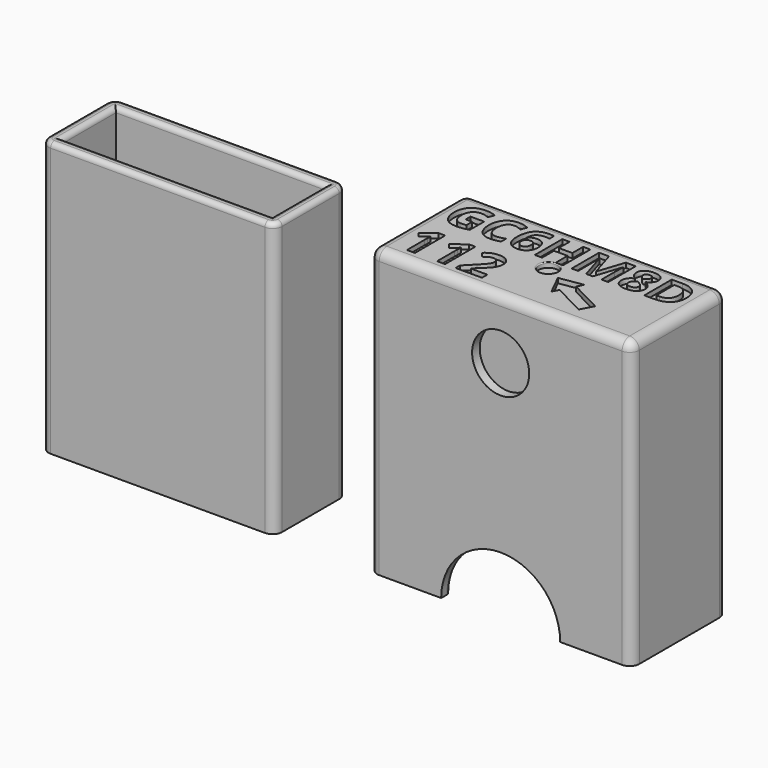
from build123d import *

# Parameters (mm, degrees)
F0_W            = 55
F0_H            = 25
F1_DEPTH        = 60
F2_T            = -2.5
F3_R            = 2
F3_TEXT_SIZE    = 10.085092972
F3_TEXT_SIZE_2  = 11.1111111111
F4_DEPTH        = 1
F5_W            = 49
F5_H            = 19
F6_DEPTH        = 57.5
F7_T            = -2.5
F9_DEPTH        = 25
F10_R           = 1
F10_2_R         = 1
F11_F1_R        = 2
F11_F2_R        = 2
F11_F3_R        = 2
F11_F4_R        = 2
F11_2_T1_DEPTH  = 62.5
F11_2_T4_ANGLE  = 90
F11_2_T6_ANGLE  = 90
F11_2_T8_ANGLE  = 90
F11_2_T10_ANGLE = 90
F12_R           = 2
F13_R           = 5
F14_DEPTH       = 2
F15_R           = 6
F16_DEPTH       = 2
F17_R           = 6
F18_DEPTH       = 2
F19_R           = 5.1
F20_DEPTH       = 1
F22_R           = 0.2
F23_DEPTH       = 1


# Not quite as in the source:
# - a fillet or chamfer that OpenCascade refuses, or shapes differently, is made with other operations: its cross-section is extruded or revolved along the edge and cut away or added
# - Text() gives the source's letters only with a copy of the font that has no kerning and outlines rounded to 1/6400 em; it was checked with that copy


with BuildPart() as f1:
    # F0 (on Top) → F1 (new body)
    with BuildSketch(Plane.XY):
        with Locations((27.5, 12.5)):
            Rectangle(F0_W, F0_H)
    extrude(amount=F1_DEPTH)

    # F2
    f2_openings = [f1.faces().sort_by_distance(p)[0] for p in [
        (27.5, 12.5, 0),
    ]]
    offset(amount=F2_T, openings=f2_openings)

    # F3 (on face) → F4 (cut)
    with BuildSketch(Plane.XY.offset(60)):
        with Locations((27.5, 12.5)):
            Circle(F3_R)
        with Locations((2.5, 14.7387330602)):
            Text('GC6HM8D', F3_TEXT_SIZE, font='Open Sans', font_style=FontStyle.BOLD, text_align=(TextAlign.LEFT, TextAlign.BOTTOM))
        with Locations((2.5, 3)):
            Text('112', F3_TEXT_SIZE_2, font='Open Sans', font_style=FontStyle.BOLD, text_align=(TextAlign.LEFT, TextAlign.BOTTOM))
    extrude(amount=-F4_DEPTH, mode=Mode.SUBTRACT)

    # F8 (on face) → F9 (cut)
    with BuildSketch(Plane(origin=(0, 25, 0), x_dir=(-1, 0, 0), z_dir=(0, 1, 0))):
        with BuildLine():
            ThreePointArc((-40, 0), (-27.5, -12.5), (-15, 0))
            Line((-15, 0), (-40, 0))
        make_face()
        with BuildLine():
            Line((-40, 0), (-15, 0))
            ThreePointArc((-15, 0), (-27.5, 12.5), (-40, 0))
        make_face()
    extrude(amount=-F9_DEPTH, mode=Mode.SUBTRACT)

    # F10#2
    f10_2_edges = [f1.edges().sort_by_distance(p)[0] for p in [
        (46.25, 2.5, 0),
        (52.5, 12.5, 0),
        (46.25, 22.5, 0),
        (8.75, 22.5, 0),
        (2.5, 12.5, 0),
        (8.75, 2.5, 0),
        (27.5, 22.5, 12.5),
        (27.5, 2.5, 12.5),
    ]]
    fillet(f10_2_edges, radius=F10_2_R)

    # F11: fillet of radius 2 on 4 edges, made by hand

    # F11_f1
    f11_f1_edges = [f1.edges().sort_by_distance(p)[0] for p in [
        (0, 25, 30),
    ]]
    fillet(f11_f1_edges, radius=F11_F1_R)

    # F11_f2
    f11_f2_edges = [f1.edges().sort_by_distance(p)[0] for p in [
        (55, 25, 30),
    ]]
    fillet(f11_f2_edges, radius=F11_F2_R)

    # F11_f3
    f11_f3_edges = [f1.edges().sort_by_distance(p)[0] for p in [
        (0, 0, 30),
    ]]
    fillet(f11_f3_edges, radius=F11_F3_R)

    # F11_f4
    f11_f4_edges = [f1.edges().sort_by_distance(p)[0] for p in [
        (55, 0, 30),
    ]]
    fillet(f11_f4_edges, radius=F11_F4_R)

    # F12
    f12_edges = [f1.edges().sort_by_distance(p)[0] for p in [
        (55, 12.5, 60),
    ]]
    fillet(f12_edges, radius=F12_R)

    # F15 (on face) → F16 (cut)
    with BuildSketch(Plane.XZ):
        with Locations((27.5, 47.5)):
            Circle(F15_R)
    extrude(amount=-F16_DEPTH, mode=Mode.SUBTRACT)

    # F17 (on face) → F18 (cut)
    with BuildSketch(Plane(origin=(0, 25, 0), x_dir=(-1, 0, 0), z_dir=(0, 1, 0))):
        with Locations((-27.5, 47.5)):
            Circle(F17_R)
    extrude(amount=-F18_DEPTH, mode=Mode.SUBTRACT)

    # F19 (on face) → F20 (cut)
    with BuildSketch(Plane(origin=(0, 0, 57.5), x_dir=(1, 0, 0), z_dir=(0, 0, -1))):
        with Locations((27.5, -12.5)):
            Circle(F19_R)
    extrude(amount=-F20_DEPTH, mode=Mode.SUBTRACT)

    # F22
    f22_edges = [f1.edges().sort_by_distance(p)[0] for p in [
        (25.5, 12.5, 60),
    ]]
    fillet(f22_edges, radius=F22_R)

    # F21 (on face) → F23 (cut)
    with BuildSketch(Plane.XY.offset(60)):
        Polygon((35.8494678515, 11.5282557422), (30.915329101, 10.7405287316), (33.1383422017, 6.2656598166), (33.8161236142, 7.581308798), (40.6146952432, 4.078896265), (41.2924766557, 5.3945452465), (41.9702580681, 6.7101942279), (35.1716864391, 10.2126067608), align=None)
    extrude(amount=-F23_DEPTH, mode=Mode.SUBTRACT)


with BuildPart() as f6:
    # F5 (on Top) → F6 (new body)
    with BuildSketch(Plane.XY):
        with Locations((-44.5, 9.5)):
            Rectangle(F5_W, F5_H)
    extrude(amount=F6_DEPTH)

    # F7
    f7_openings = [f6.faces().sort_by_distance(p)[0] for p in [
        (-44.5, 9.5, 57.5),
    ]]
    offset(amount=F7_T, openings=f7_openings)

    # F10
    f10_edges = [f6.edges().sort_by_distance(p)[0] for p in [
        (-44.5, 0, 57.5),
        (-20, 9.5, 57.5),
        (-44.5, 19, 57.5),
        (-69, 9.5, 57.5),
        (-44.5, 2.5, 57.5),
        (-66.5, 9.5, 57.5),
        (-44.5, 16.5, 57.5),
        (-22.5, 9.5, 57.5),
    ]]
    fillet(f10_edges, radius=F10_R)

    # F11#2: fillet of radius 2 on 4 edges, made by hand

    # F11_2_s2 → F11_2_t1 (cut)
    with BuildSketch(Plane.XY.offset(-5)):
        with BuildLine():
            ThreePointArc((-67, 0), (-68.4142135624, 0.5857864376), (-69, 2))
            Line((-69, 2), (-69, 0))
            Line((-69, 0), (-67, 0))
        make_face()
        with BuildLine():
            ThreePointArc((-69, 17), (-68.4142135624, 18.4142135624), (-67, 19))
            Line((-67, 19), (-69, 19))
            Line((-69, 19), (-69, 17))
        make_face()
        with BuildLine():
            ThreePointArc((-22, 0), (-20.5857864376, 0.5857864376), (-20, 2))
            Line((-20, 2), (-20, 0))
            Line((-20, 0), (-22, 0))
        make_face()
        with BuildLine():
            ThreePointArc((-20, 17), (-20.5857864376, 18.4142135624), (-22, 19))
            Line((-22, 19), (-20, 19))
            Line((-20, 19), (-20, 17))
        make_face()
    extrude(amount=F11_2_T1_DEPTH, mode=Mode.SUBTRACT)

    # F11_2_s3 → F11_2_t4 (revolve, cut)
    with BuildSketch(Plane.XZ.offset(-17)):
        with BuildLine():
            ThreePointArc((-21, 57.5), (-20.2928932188, 57.2071067812), (-20, 56.5))
            Line((-20, 56.5), (-20, 57.5))
            Line((-20, 57.5), (-21, 57.5))
        make_face()
    revolve(axis=Axis((-22, 17, 57.5), (0, 0, 1)), revolution_arc=F11_2_T4_ANGLE, mode=Mode.SUBTRACT)

    # F11_2_s5 → F11_2_t6 (revolve, cut)
    with BuildSketch(Plane.YZ.offset(-22)):
        with BuildLine():
            ThreePointArc((1, 57.5), (0.2928932188, 57.2071067812), (0, 56.5))
            Line((0, 56.5), (0, 57.5))
            Line((0, 57.5), (1, 57.5))
        make_face()
    revolve(axis=Axis((-22, 2, 57.5), (0, 0, 1)), revolution_arc=F11_2_T6_ANGLE, mode=Mode.SUBTRACT)

    # F11_2_s7 → F11_2_t8 (revolve, cut)
    with BuildSketch(Plane.YZ.offset(-67)):
        with BuildLine():
            ThreePointArc((18, 57.5), (18.7071067812, 57.2071067812), (19, 56.5))
            Line((19, 56.5), (19, 57.5))
            Line((19, 57.5), (18, 57.5))
        make_face()
    revolve(axis=Axis((-67, 17, 57.5), (0, 0, 1)), revolution_arc=F11_2_T8_ANGLE, mode=Mode.SUBTRACT)

    # F11_2_s9 → F11_2_t10 (revolve, cut)
    with BuildSketch(Plane.XZ.offset(-2)):
        with BuildLine():
            ThreePointArc((-68, 57.5), (-68.7071067812, 57.2071067812), (-69, 56.5))
            Line((-69, 56.5), (-69, 57.5))
            Line((-69, 57.5), (-68, 57.5))
        make_face()
    revolve(axis=Axis((-67, 2, 57.5), (0, 0, 1)), revolution_arc=F11_2_T10_ANGLE, mode=Mode.SUBTRACT)

    # F13 (on face) → F14 (cut)
    with BuildSketch(Plane(origin=(0, 2.5, 0), x_dir=(-1, 0, 0), z_dir=(0, 1, 0))):
        with Locations((44.5, 47.5)):
            Circle(F13_R)
    extrude(amount=-F14_DEPTH, mode=Mode.SUBTRACT)


solid = Compound([f1.part, f6.part])
